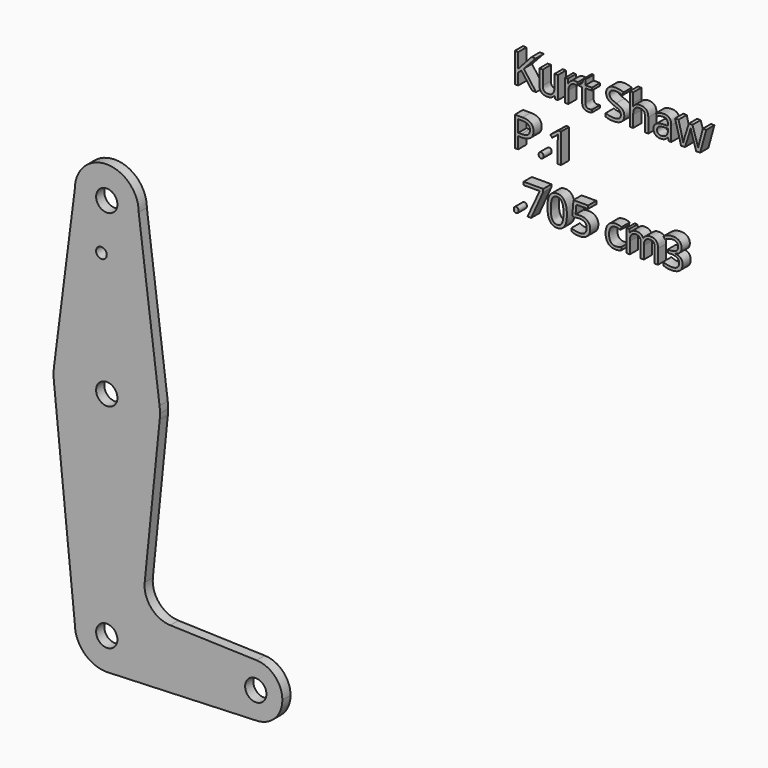
from build123d import *

# Parameters (mm, degrees)
F0_R         = 3.175
F0_R_2       = 1.5875
F0_TEXT_SIZE = 12.3204249475
F1_DEPTH     = 3.048


# Not quite as in the source:
# - Text() gives the source's letters only with a copy of the font that has no kerning and outlines rounded to 1/6400 em; it was checked with that copy


with BuildPart() as f1:
    # F0 (on Front) → F1 (new body)
    with BuildSketch(Plane.XZ):
        with BuildLine():
            ThreePointArc((-9.525, 50.8), (0, 41.275), (9.525, 50.8))
            ThreePointArc((9.525, 50.8), (0, 60.325), (-9.525, 50.8))
        make_face()
        with Locations((0, 50.8)):
            Circle(F0_R, mode=Mode.SUBTRACT)
        with BuildLine():
            Line((15.7474569047, 2.0082893304), (9.525, 50.8))
            ThreePointArc((9.525, 50.8), (0, 41.275), (-9.525, 50.8))
            Line((-9.525, 50.8), (-15.7474569047, 2.0082893304))
            ThreePointArc((-15.7474569047, 2.0082893304), (0, 15.875), (15.7474569047, 2.0082893304))
        make_face()
        with Locations((-1.5875, 36.5252)):
            Circle(F0_R_2, mode=Mode.SUBTRACT)
        with BuildLine():
            ThreePointArc((15.875, 0), (15.8430821396, 1.0061676396), (15.7474569047, 2.0082893304))
            ThreePointArc((15.7474569047, 2.0082893304), (0, 15.875), (-15.7474569047, 2.0082893304))
            ThreePointArc((-15.7474569047, 2.0082893304), (-15.873667691, 0.2056672947), (-15.7942028036, -1.5996195795))
            ThreePointArc((-15.7942028036, -1.5996195795), (-0.0004482141, -15.8749999937), (15.7941124512, -1.6005114426))
            ThreePointArc((15.7941124512, -1.6005114426), (15.8547652169, -0.8012770547), (15.875, 0))
        make_face()
        Circle(F0_R, mode=Mode.SUBTRACT)
        with BuildLine():
            ThreePointArc((15.7941124512, -1.6005114426), (-0.0004482141, -15.8749999937), (-15.7942028036, -1.5996195795))
            Line((-15.7942028036, -1.5996195795), (-9.525, -63.5))
            ThreePointArc((-9.525, -63.5), (0, -53.975), (9.525, -63.5))
            ThreePointArc((9.525, -63.5), (6.9936612334, -69.9663998912), (0.7450887029, -72.9958131734))
            Line((0.7450887029, -72.9958131734), (44.7604045361, -71.2716327043))
            ThreePointArc((44.7604045361, -71.2716327043), (36.5122633209, -63.3685325333), (44.7038065708, -55.4067836673))
            Line((44.7038065708, -55.4067836673), (18.9667787686, -54.582472297))
            ThreePointArc((18.9667787686, -54.582472297), (13.2384784959, -51.8719726214), (11.3115875631, -45.8348107188))
            Line((11.3115875631, -45.8348107188), (15.7941124512, -1.6005114426))
        make_face()
        with BuildLine():
            ThreePointArc((9.525, -63.5), (0, -53.975), (-9.525, -63.5))
            ThreePointArc((-9.525, -63.5), (-6.7351920908, -70.2351920908), (0, -73.025))
            Line((0, -73.025), (0.7450887029, -72.9958131734))
            ThreePointArc((0.7450887029, -72.9958131734), (6.9936612334, -69.9663998912), (9.525, -63.5))
        make_face()
        with Locations((0, -63.5)):
            Circle(F0_R, mode=Mode.SUBTRACT)
        with BuildLine():
            Line((0.7450887029, -72.9958131734), (0, -73.025))
            ThreePointArc((0, -73.025), (0.3728300705, -73.0177004964), (0.7450887029, -72.9958131734))
        make_face()
        with BuildLine():
            ThreePointArc((52.3872128107, -63.340215624), (50.1515009281, -57.8181219527), (44.7038065708, -55.4067836673))
            ThreePointArc((44.7038065708, -55.4067836673), (36.5122633209, -63.3685325333), (44.7604045361, -71.2716327043))
            ThreePointArc((44.7604045361, -71.2716327043), (50.1711646291, -68.841933114), (52.3872128107, -63.340215624))
        make_face()
        with Locations((44.4497128107, -63.340215624)):
            Circle(F0_R, mode=Mode.SUBTRACT)
        with Locations((120.5220595002, 120.9217905998)):
            Text('Kurt Shaw', F0_TEXT_SIZE, font='Open Sans', text_align=(TextAlign.LEFT, TextAlign.BOTTOM))
        with Locations((120.5220595002, 104.1660126713)):
            Text('P.1', F0_TEXT_SIZE, font='Open Sans', text_align=(TextAlign.LEFT, TextAlign.BOTTOM))
        with Locations((120.5220595002, 87.4102347427)):
            Text('.705 cm3', F0_TEXT_SIZE, font='Open Sans', text_align=(TextAlign.LEFT, TextAlign.BOTTOM))
    extrude(amount=F1_DEPTH)


solid = f1.part
